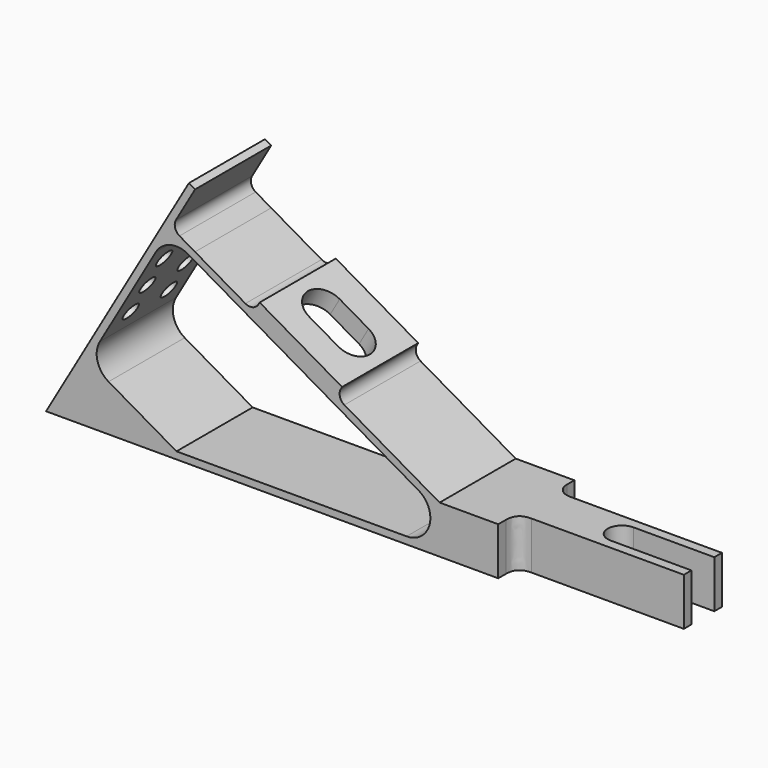
from build123d import *

# Parameters (mm, degrees)
F1_DEPTH    = 20
F2_W        = 35
F2_H        = 10
F3_DEPTH    = 5
F4_W        = 35
F4_H        = 10
F5_DEPTH    = 5
F7_DEPTH    = 25
F8_T1_DEPTH = 10
F9_R        = 3
F10_R       = 2
F11_R       = 2
F12_R       = 2
F14_DEPTH   = 15
F15_R       = 5.5
F16_DEPTH   = 2
F17_R       = 4.25
F18_DEPTH   = 110.5843026286
F19_R       = 1.8416313508
F20_DEPTH   = 10


# Not quite as in the source:
# - a fillet or chamfer that OpenCascade refuses, or shapes differently, is made with other operations: its cross-section is extruded or revolved along the edge and cut away or added


with BuildPart() as f1:
    # F0 (on Front) → F1 (new body)
    with BuildSketch(Plane.XZ):
        Polygon((48.965709947, 58.1432288134), (47.6666718414, 58.8932288134), (17.6666718414, 6.9317045863), (147.6666718414, 6.9317045863), (147.6666718414, 16.9317045863), (100.3461637657, 16.9317045863), (78.6067260984, 29.4829747755), (79.8567260984, 31.648038285), (62.5362180227, 41.648038285), (61.2862180227, 39.4829747755), (48.965709947, 46.5962234296), (43.965709947, 49.4829747755), align=None)
        with BuildLine():
            Line((45.06859563, 8.4317045863), (30.795836966, 16.6720856431))
            ThreePointArc((30.795836966, 16.6720856431), (28.4662078345, 19.7081174365), (28.965709947, 23.502212662))
            Line((28.965709947, 23.502212662), (40.715709947, 43.8538096509))
            ThreePointArc((40.715709947, 43.8538096509), (43.7517417405, 46.1834387824), (47.545836966, 45.6839366698))
            Line((47.545836966, 45.6839366698), (95.9083415922, 17.7618316052))
            ThreePointArc((95.9083415922, 17.7618316052), (98.2379707236, 12.1376093608), (93.4083415922, 8.4317045863))
            Line((93.4083415922, 8.4317045863), (45.06859563, 8.4317045863))
        make_face(mode=Mode.SUBTRACT)
    extrude(amount=F1_DEPTH)

    # F2 (on face) → F3 (cut)
    with BuildSketch(Plane.XZ.offset(20)):
        with Locations((130.1666718414, 11.9317045863)):
            Rectangle(F2_W, F2_H)
    extrude(amount=-F3_DEPTH, mode=Mode.SUBTRACT)

    # F4 (on face) → F5 (cut)
    with BuildSketch(Plane(origin=(0, 0, 0), x_dir=(-1, 0, 0), z_dir=(0, 1, 0))):
        with Locations((-130.1666718414, 11.9317045863)):
            Rectangle(F4_W, F4_H)
    extrude(amount=-F5_DEPTH, mode=Mode.SUBTRACT)

    # F6 (on face) → F7 (cut)
    with BuildSketch(Plane.XY.offset(16.9317045863)):
        with BuildLine():
            Line((147.6666718414, -7.0000102813), (130.6745260024, -7.0000102813))
            ThreePointArc((130.6745260024, -7.0000102813), (130.6666718414, -7), (130.6588176804, -7.0000102813))
            ThreePointArc((130.6588176804, -7.0000102813), (127.6666744117, -10.0039270839), (130.6666718414, -13))
            Line((130.6666718414, -13), (147.6666718414, -13))
            Line((147.6666718414, -13), (147.6666718414, -7.0000102813))
        make_face()
    extrude(amount=-F7_DEPTH, mode=Mode.SUBTRACT)

    # F8: fillet of radius 3 on 1 edges, made by hand

    # F8_s2 → F8_t1 (join)
    with BuildSketch(Plane.XY.offset(6.9317045863)):
        with BuildLine():
            add(Edge.make_bspline(
                [(112.6666718414, -18), (112.6666718414, -15), (115.6666718414, -15)],
                knots=[0, 0, 0, 1, 1, 1], degree=2, weights=[1, 1, 1]))
            Line((115.6666718414, -15), (112.6666718414, -15))
            Line((112.6666718414, -15), (112.6666718414, -18))
        make_face()
    extrude(amount=F8_T1_DEPTH)

    # F9
    f9_edges = [f1.edges().sort_by_distance(p)[0] for p in [
        (112.666672, -5, 11.931705),
    ]]
    fillet(f9_edges, radius=F9_R)

    # F10
    f10_edges = [f1.edges().sort_by_distance(p)[0] for p in [
        (78.606726, -10, 29.482975),
    ]]
    fillet(f10_edges, radius=F10_R)

    # F11
    f11_edges = [f1.edges().sort_by_distance(p)[0] for p in [
        (61.286218, -10, 39.482975),
    ]]
    fillet(f11_edges, radius=F11_R)

    # F12
    f12_edges = [f1.edges().sort_by_distance(p)[0] for p in [
        (43.96571, -10, 49.482975),
    ]]
    fillet(f12_edges, radius=F12_R)

    # F13 (on face) → F14 (cut)
    with BuildSketch(Plane(origin=(33.668184092, 0, 58.3150054459), x_dir=(0.8660254038, 0, -0.5), z_dir=(0.5, 0, 0.8660254038))):
        with BuildLine():
            Line((46.8339343218, -6), (39.8339343218, -6))
            ThreePointArc((39.8339343218, -6), (35.8339343218, -10), (39.8339343218, -14))
            Line((39.8339343218, -14), (46.8339343218, -14))
            ThreePointArc((46.8339343218, -14), (50.8339343218, -10), (46.8339343218, -6))
        make_face()
    extrude(amount=-F14_DEPTH, mode=Mode.SUBTRACT)

    # F15 (on face) → F16 (cut)
    with BuildSketch(Plane(origin=(10.2484877494, 0, -5.9169671609), x_dir=(0, -1, 0), z_dir=(-0.8660254038, 0, 0.5))):
        with Locations((10, 22.3363681839)):
            Circle(F15_R)
    extrude(amount=-F16_DEPTH, mode=Mode.SUBTRACT)

    # F17 (on face) → F18 (cut, through all)
    with BuildSketch(Plane(origin=(11.980538557, 0, -6.9169671609), x_dir=(0, -1, 0), z_dir=(-0.8660254038, 0, 0.5))):
        with Locations((10, 22.3363681839)):
            Circle(F17_R)
    extrude(amount=-F18_DEPTH, mode=Mode.SUBTRACT)

    # F19 (on face) → F20 (cut)
    with BuildSketch(Plane(origin=(10.2484877494, 0, -5.9169671609), x_dir=(0, -1, 0), z_dir=(-0.8660254038, 0, 0.5))):
        with Locations((15, 53.8363681839)):
            Circle(F19_R)
        with Locations((5, 53.8363681839)):
            Circle(F19_R)
        with Locations((5, 46.8363681839)):
            Circle(F19_R)
        with Locations((15, 46.8363681839)):
            Circle(F19_R)
        with Locations((15, 39.8363681839)):
            Circle(F19_R)
        with Locations((5, 39.8363681839)):
            Circle(F19_R)
    extrude(amount=-F20_DEPTH, mode=Mode.SUBTRACT)


solid = f1.part
